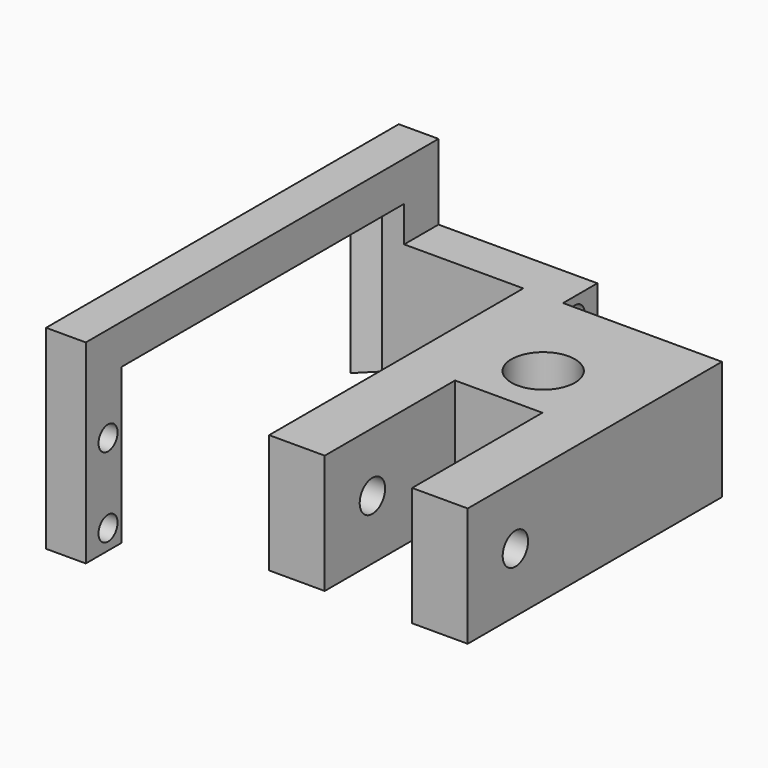
from build123d import *

# Parameters (mm, degrees)
F0_R         = 4
F1_DEPTH     = 15
F3_W         = 15
F3_H         = 15
F3_R         = 2
F4_DEPTH     = 7
F6_W         = 15
F6_H         = 15
F6_R         = 2
F7_DEPTH     = 7
F8_W         = 5.4
F8_H         = 15
F8_R         = 1.5
F9_DEPTH     = 5
F10_DEPTH    = 20
F12_W        = 5.4
F12_H        = 2.5
F12_W_2      = 7.6
F12_H_2      = 15
F12_R        = 1.5
F13_DEPTH    = 5
F12_W_3      = 2.2
F12_H_3      = 2
F14_DEPTH    = 3
F15_T4_DEPTH = 27.2150489639
F16_SIZE     = 2


# Not quite as in the source:
# - a fillet or chamfer that OpenCascade refuses, or shapes differently, is made with other operations: its cross-section is extruded or revolved along the edge and cut away or added


with BuildPart() as f1:
    # F0 (on Top) → F1 (new body)
    with BuildSketch(Plane.XY):
        Polygon((12.5, -12.5), (12.5, 12.5), (-12.5, 12.5), (-12.5, -12.5), (-5.5, -12.5), (-5.5, -7), (5.5, -7), (5.5, -12.5), align=None)
        Circle(F0_R, mode=Mode.SUBTRACT)
    extrude(amount=F1_DEPTH)

    # F3 (on offset) → F4 (join)
    with BuildSketch(Plane(origin=(-12.5, 0, 0), x_dir=(0, -1, 0), z_dir=(-1, 0, 0))):
        with Locations((20, 7.5)):
            Rectangle(F3_W, F3_H)
        with Locations((20, 7.5)):
            Circle(F3_R, mode=Mode.SUBTRACT)
    extrude(amount=-F4_DEPTH)

    # F6 (on offset) → F7 (join)
    with BuildSketch(Plane.YZ.offset(12.5)):
        with Locations((-20, 7.5)):
            Rectangle(F6_W, F6_H)
        with Locations((-20, 7.5)):
            Circle(F6_R, mode=Mode.SUBTRACT)
    extrude(amount=-F7_DEPTH)

    # F8 (on offset) → F9 (join)
    with BuildSketch(Plane(origin=(-12.5, 0, 0), x_dir=(0, -1, 0), z_dir=(-1, 0, 0))):
        with Locations((-15.2, 7.5)):
            Rectangle(F8_W, F8_H)
        with Locations((-14.4, 2.5)):
            Circle(F8_R, mode=Mode.SUBTRACT)
        with Locations((-14.4, 12.5)):
            Circle(F8_R, mode=Mode.SUBTRACT)
    extrude(amount=-F9_DEPTH)

    # F8 (on offset) → F10 (join)
    with BuildSketch(Plane(origin=(-12.5, 0, 0), x_dir=(0, -1, 0), z_dir=(-1, 0, 0))):
        with Locations((-15.2, 7.5)):
            Rectangle(F8_W, F8_H)
        with Locations((-14.4, 2.5)):
            Circle(F8_R, mode=Mode.SUBTRACT)
        with Locations((-14.4, 12.5)):
            Circle(F8_R, mode=Mode.SUBTRACT)
    extrude(amount=F10_DEPTH)

    # F12 (on offset) → F13 (join)
    with BuildSketch(Plane(origin=(-32.5, 0, 0), x_dir=(0, -1, 0), z_dir=(-1, 0, 0))):
        with Locations((-15.2, 16.25)):
            Rectangle(F12_W, F12_H)
        Polygon((30, 19.5), (30, 17.5), (37.6, 17.5), (37.6, 24.5), (-17.9, 24.5), (-17.9, 17.5), (-12.5, 17.5), (-12.5, 19.5), (-10.3, 19.5), align=None)
        with Locations((33.8, 16.25)):
            Rectangle(F12_W_2, F12_H)
        with Locations((33.8, 7.5)):
            Rectangle(F12_W_2, F12_H_2)
        with Locations((34.1, 2.5)):
            Circle(F12_R, mode=Mode.SUBTRACT)
        with Locations((34.1, 12.5)):
            Circle(F12_R, mode=Mode.SUBTRACT)
    extrude(amount=-F13_DEPTH)

    # F12 (on offset) → F14 (join)
    with BuildSketch(Plane(origin=(-32.5, 0, 0), x_dir=(0, -1, 0), z_dir=(-1, 0, 0))):
        with Locations((-11.4, 7.5)):
            Rectangle(F12_W_3, F12_H_2)
        with Locations((-11.4, 16.25)):
            Rectangle(F12_W_3, F12_H)
        with Locations((-11.4, 18.5)):
            Rectangle(F12_W_3, F12_H_3)
    extrude(amount=-F14_DEPTH)

    # F15: chamfer of 3 on 1 edges, made by hand


with BuildPart() as f15_tool2:
    # F15_s3 → F15_t4 (new body)
    with BuildSketch(Plane.XY.offset(-7.7150489639)):
        Polygon((-29.5, 13.3), (-32.5, 10.3), (-29.5, 10.3), align=None)
    extrude(amount=F15_T4_DEPTH)

    split(bisect_by=Plane.XZ.offset(-12.5), keep=Keep.TOP)


with BuildPart() as f1_1:
    add(f1.part)

    # F15_t1: cut F15_tool2
    add(f15_tool2.part, mode=Mode.SUBTRACT)

    # F16
    f16_edges = [f1_1.edges().sort_by_distance(p)[0] for p in [
        (-27.5, -30, 9.75),
    ]]
    chamfer(f16_edges, length=F16_SIZE)


solid = f1_1.part
